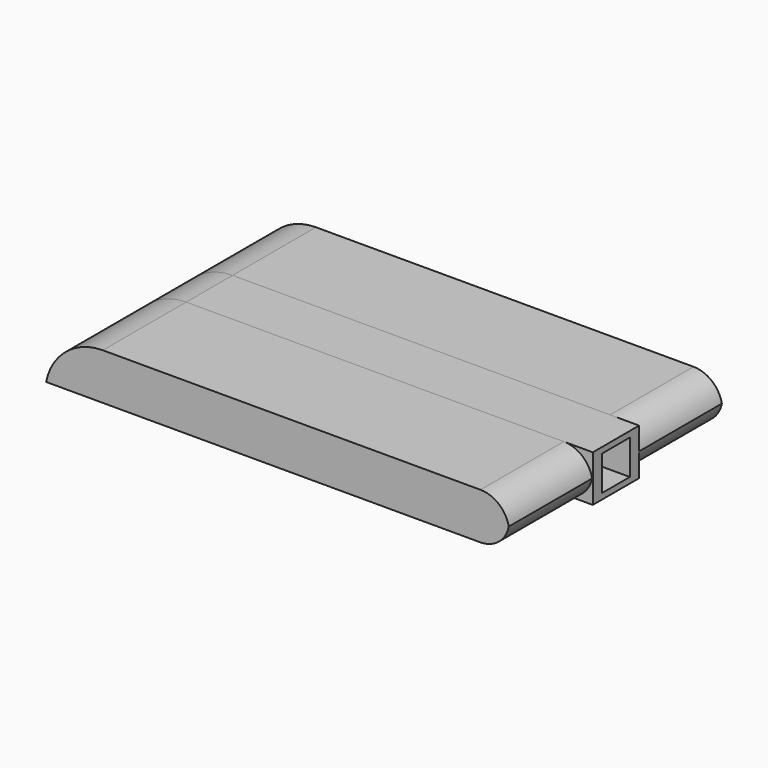
from build123d import *

# Parameters (mm, degrees)
F0_W          = 9
F0_H          = 4
F1_DEPTH      = 40
F0_W_2        = 5
F2_DEPTH      = 40
F3_W          = 3
F3_H          = 3
F4_DEPTH      = 10
F5_T1_DEPTH   = 33.4948974279
F5_2_T1_DEPTH = 33.4948974279
F5_3_T1_DEPTH = 29.4948974279
F6_T1_DEPTH   = 21.5
F6_2_T1_DEPTH = 21.5


# Not quite as in the source:
# - a fillet or chamfer that OpenCascade refuses, or shapes differently, is made with other operations: its cross-section is extruded or revolved along the edge and cut away or added


with BuildPart() as f1:
    # F0 (on Right) → F1 (new body)
    with BuildSketch(Plane.YZ):
        with Locations((-4.5, 2)):
            Rectangle(F0_W, F0_H)
    extrude(amount=F1_DEPTH)

    # F5: fillet of radius 5 on 1 edges, made by hand

    # F5_s2 → F5_t1 (cut)
    with BuildSketch(Plane.XZ.offset(-12.2474487139)):
        with BuildLine():
            ThreePointArc((4.8989794856, 4), (1.7367018254, 2.8729833462), (0, 0))
            Line((0, 0), (0, 4))
            Line((0, 4), (4.8989794856, 4))
        make_face()
    extrude(amount=F5_T1_DEPTH, mode=Mode.SUBTRACT)

    # F6: fillet of radius 2.5 on 2 edges, made by hand

    # F6_s2 → F6_t1 (cut)
    with BuildSketch(Plane.XZ.offset(-6.25)):
        with BuildLine():
            ThreePointArc((40, 1.5), (39.267766953, 3.267766953), (37.5, 4))
            Line((37.5, 4), (40, 4))
            Line((40, 4), (40, 1.5))
        make_face()
        with BuildLine():
            ThreePointArc((37.5, 0), (39.267766953, 0.732233047), (40, 2.5))
            Line((40, 2.5), (40, 0))
            Line((40, 0), (37.5, 0))
        make_face()
    extrude(amount=F6_T1_DEPTH, mode=Mode.SUBTRACT)


with BuildPart() as f1b:
    # F0 (on Right) → F1, piece 2 (new body)
    with BuildSketch(Plane.YZ):
        with Locations((9.5, 2)):
            Rectangle(F0_W, F0_H)
    extrude(amount=F1_DEPTH)

    # F5#2: fillet of radius 5 on 1 edges, made by hand

    # F5_2_s2 → F5_2_t1 (cut)
    with BuildSketch(Plane.XZ.offset(-26.2474487139)):
        with BuildLine():
            ThreePointArc((4.8989794856, 4), (1.7367018254, 2.8729833462), (0, 0))
            Line((0, 0), (0, 4))
            Line((0, 4), (4.8989794856, 4))
        make_face()
    extrude(amount=F5_2_T1_DEPTH, mode=Mode.SUBTRACT)

    # F6#2: fillet of radius 2.5 on 2 edges, made by hand

    # F6_2_s2 → F6_2_t1 (cut)
    with BuildSketch(Plane.XZ.offset(-20.25)):
        with BuildLine():
            ThreePointArc((40, 1.5), (39.267766953, 3.267766953), (37.5, 4))
            Line((37.5, 4), (40, 4))
            Line((40, 4), (40, 1.5))
        make_face()
        with BuildLine():
            ThreePointArc((37.5, 0), (39.267766953, 0.732233047), (40, 2.5))
            Line((40, 2.5), (40, 0))
            Line((40, 0), (37.5, 0))
        make_face()
    extrude(amount=F6_2_T1_DEPTH, mode=Mode.SUBTRACT)


with BuildPart() as f2:
    # F0 (on Right) → F2 (new body)
    with BuildSketch(Plane.YZ):
        with Locations((2.5, 2)):
            Rectangle(F0_W_2, F0_H)
    extrude(amount=F2_DEPTH)

    # F3 (on face) → F4 (cut)
    with BuildSketch(Plane.YZ.offset(40)):
        with Locations((2.5, 2)):
            Rectangle(F3_W, F3_H)
    extrude(amount=-F4_DEPTH, mode=Mode.SUBTRACT)

    # F5#3: fillet of radius 5 on 1 edges, made by hand

    # F5_3_s2 → F5_3_t1 (cut)
    with BuildSketch(Plane.XZ.offset(-17.2474487139)):
        with BuildLine():
            ThreePointArc((4.8989794856, 4), (1.7367018254, 2.8729833462), (0, 0))
            Line((0, 0), (0, 4))
            Line((0, 4), (4.8989794856, 4))
        make_face()
    extrude(amount=F5_3_T1_DEPTH, mode=Mode.SUBTRACT)


solid = Compound([f1.part, f1b.part, f2.part])
